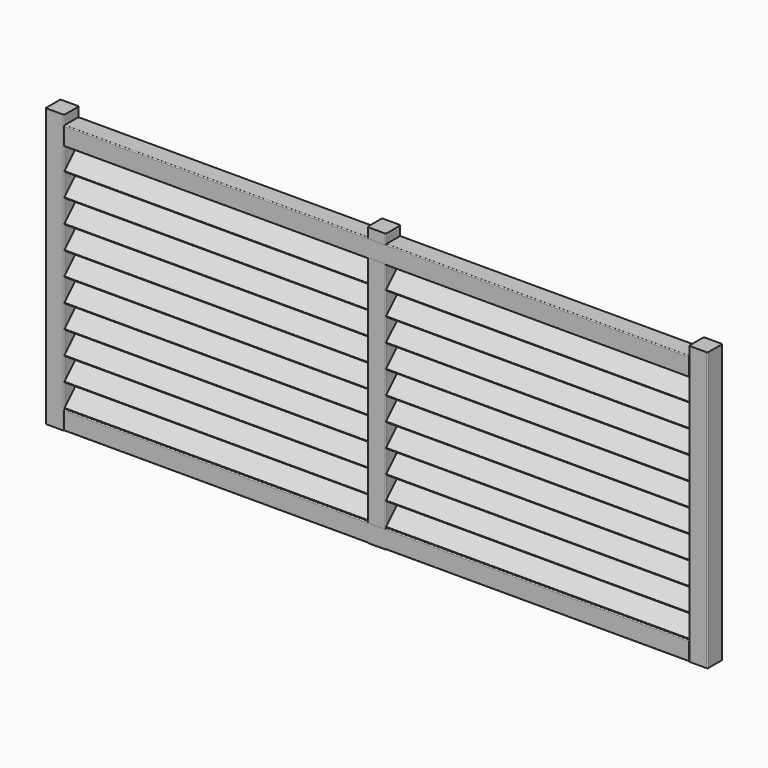
from build123d import *

# Parameters (mm, degrees)
F1_DEPTH      = 3370
F3_DEPTH      = 1400
F3_DEPTH_BACK = 100
F4_W          = 90
F4_H          = 100
F5_DEPTH      = 3370


# Not quite as in the source:
# - a feature names something its author has since deleted; it is built from what else it names


with BuildPart() as f1:
    # F0 (on Right) → F1 (new body)
    with BuildSketch(Plane.YZ):
        with BuildLine():
            ThreePointArc((-1.4142135624, 1.4142135624), (0, 0.8284271247), (1.4142135624, 1.4142135624))
            Line((1.4142135624, 1.4142135624), (89.8025612107, 89.8025612107))
            ThreePointArc((89.8025612107, 89.8025612107), (90.3883476483, 91.2167747731), (89.8025612107, 92.6309883354))
            Line((89.8025612107, 92.6309883354), (85.5599205236, 96.8736290226))
            ThreePointArc((85.5599205236, 96.8736290226), (84.1457069612, 97.4594154602), (82.7314933988, 96.8736290226))
            Line((82.7314933988, 96.8736290226), (-5.6568542495, 8.4852813742))
            ThreePointArc((-5.6568542495, 8.4852813742), (-6.2426406871, 7.0710678119), (-5.6568542495, 5.6568542495))
            Line((-5.6568542495, 5.6568542495), (-1.4142135624, 1.4142135624))
        make_face()
    extrude(amount=F1_DEPTH)


with BuildPart() as f1b:
    # F0 (on Right) → F1, piece 2 (new body)
    with BuildSketch(Plane.YZ):
        with BuildLine():
            ThreePointArc((-1.4142135624, 126.4142135624), (0, 125.8284271247), (1.4142135624, 126.4142135624))
            Line((1.4142135624, 126.4142135624), (89.8025612107, 214.8025612107))
            ThreePointArc((89.8025612107, 214.8025612107), (90.3883476483, 216.2167747731), (89.8025612107, 217.6309883354))
            Line((89.8025612107, 217.6309883354), (85.5599205236, 221.8736290226))
            ThreePointArc((85.5599205236, 221.8736290226), (84.1457069612, 222.4594154602), (82.7314933988, 221.8736290226))
            Line((82.7314933988, 221.8736290226), (-5.6568542495, 133.4852813742))
            ThreePointArc((-5.6568542495, 133.4852813742), (-6.2426406871, 132.0710678119), (-5.6568542495, 130.6568542495))
            Line((-5.6568542495, 130.6568542495), (-1.4142135624, 126.4142135624))
        make_face()
    extrude(amount=F1_DEPTH)


with BuildPart() as f1c:
    # F0 (on Right) → F1, piece 3 (new body)
    with BuildSketch(Plane.YZ):
        with BuildLine():
            ThreePointArc((-1.4142135624, 251.4142135624), (0, 250.8284271247), (1.4142135624, 251.4142135624))
            Line((1.4142135624, 251.4142135624), (89.8025612107, 339.8025612107))
            ThreePointArc((89.8025612107, 339.8025612107), (90.3883476483, 341.2167747731), (89.8025612107, 342.6309883354))
            Line((89.8025612107, 342.6309883354), (85.5599205236, 346.8736290226))
            ThreePointArc((85.5599205236, 346.8736290226), (84.1457069612, 347.4594154602), (82.7314933988, 346.8736290226))
            Line((82.7314933988, 346.8736290226), (-5.6568542495, 258.4852813742))
            ThreePointArc((-5.6568542495, 258.4852813742), (-6.2426406871, 257.0710678119), (-5.6568542495, 255.6568542495))
            Line((-5.6568542495, 255.6568542495), (-1.4142135624, 251.4142135624))
        make_face()
    extrude(amount=F1_DEPTH)


with BuildPart() as f1d:
    # F0 (on Right) → F1, piece 4 (new body)
    with BuildSketch(Plane.YZ):
        with BuildLine():
            ThreePointArc((-1.4142135624, 376.4142135624), (0, 375.8284271247), (1.4142135624, 376.4142135624))
            Line((1.4142135624, 376.4142135624), (89.8025612107, 464.8025612107))
            ThreePointArc((89.8025612107, 464.8025612107), (90.3883476483, 466.2167747731), (89.8025612107, 467.6309883354))
            Line((89.8025612107, 467.6309883354), (85.5599205236, 471.8736290226))
            ThreePointArc((85.5599205236, 471.8736290226), (84.1457069612, 472.4594154602), (82.7314933988, 471.8736290226))
            Line((82.7314933988, 471.8736290226), (-5.6568542495, 383.4852813742))
            ThreePointArc((-5.6568542495, 383.4852813742), (-6.2426406871, 382.0710678119), (-5.6568542495, 380.6568542495))
            Line((-5.6568542495, 380.6568542495), (-1.4142135624, 376.4142135624))
        make_face()
    extrude(amount=F1_DEPTH)


with BuildPart() as f1e:
    # F0 (on Right) → F1, piece 5 (new body)
    with BuildSketch(Plane.YZ):
        with BuildLine():
            ThreePointArc((-1.4142135624, 501.4142135624), (0, 500.8284271247), (1.4142135624, 501.4142135624))
            Line((1.4142135624, 501.4142135624), (89.8025612107, 589.8025612107))
            ThreePointArc((89.8025612107, 589.8025612107), (90.3883476483, 591.2167747731), (89.8025612107, 592.6309883354))
            Line((89.8025612107, 592.6309883354), (85.5599205236, 596.8736290226))
            ThreePointArc((85.5599205236, 596.8736290226), (84.1457069612, 597.4594154602), (82.7314933988, 596.8736290226))
            Line((82.7314933988, 596.8736290226), (-5.6568542495, 508.4852813742))
            ThreePointArc((-5.6568542495, 508.4852813742), (-6.2426406871, 507.0710678119), (-5.6568542495, 505.6568542495))
            Line((-5.6568542495, 505.6568542495), (-1.4142135624, 501.4142135624))
        make_face()
    extrude(amount=F1_DEPTH)


with BuildPart() as f1f:
    # F0 (on Right) → F1, piece 6 (new body)
    with BuildSketch(Plane.YZ):
        with BuildLine():
            ThreePointArc((-1.4142135624, 626.4142135624), (0, 625.8284271247), (1.4142135624, 626.4142135624))
            Line((1.4142135624, 626.4142135624), (89.8025612107, 714.8025612107))
            ThreePointArc((89.8025612107, 714.8025612107), (90.3883476483, 716.2167747731), (89.8025612107, 717.6309883354))
            Line((89.8025612107, 717.6309883354), (85.5599205236, 721.8736290226))
            ThreePointArc((85.5599205236, 721.8736290226), (84.1457069612, 722.4594154602), (82.7314933988, 721.8736290226))
            Line((82.7314933988, 721.8736290226), (-5.6568542495, 633.4852813742))
            ThreePointArc((-5.6568542495, 633.4852813742), (-6.2426406871, 632.0710678119), (-5.6568542495, 630.6568542495))
            Line((-5.6568542495, 630.6568542495), (-1.4142135624, 626.4142135624))
        make_face()
    extrude(amount=F1_DEPTH)


with BuildPart() as f1g:
    # F0 (on Right) → F1, piece 7 (new body)
    with BuildSketch(Plane.YZ):
        with BuildLine():
            ThreePointArc((-1.4142135624, 751.4142135624), (0, 750.8284271247), (1.4142135624, 751.4142135624))
            Line((1.4142135624, 751.4142135624), (89.8025612107, 839.8025612107))
            ThreePointArc((89.8025612107, 839.8025612107), (90.3883476483, 841.2167747731), (89.8025612107, 842.6309883354))
            Line((89.8025612107, 842.6309883354), (85.5599205236, 846.8736290226))
            ThreePointArc((85.5599205236, 846.8736290226), (84.1457069612, 847.4594154602), (82.7314933988, 846.8736290226))
            Line((82.7314933988, 846.8736290226), (-5.6568542495, 758.4852813742))
            ThreePointArc((-5.6568542495, 758.4852813742), (-6.2426406871, 757.0710678119), (-5.6568542495, 755.6568542495))
            Line((-5.6568542495, 755.6568542495), (-1.4142135624, 751.4142135624))
        make_face()
    extrude(amount=F1_DEPTH)


with BuildPart() as f1h:
    # F0 (on Right) → F1, piece 8 (new body)
    with BuildSketch(Plane.YZ):
        with BuildLine():
            ThreePointArc((-1.4142135624, 876.4142135624), (0, 875.8284271247), (1.4142135624, 876.4142135624))
            Line((1.4142135624, 876.4142135624), (89.8025612107, 964.8025612107))
            ThreePointArc((89.8025612107, 964.8025612107), (90.3883476483, 966.2167747731), (89.8025612107, 967.6309883354))
            Line((89.8025612107, 967.6309883354), (85.5599205236, 971.8736290226))
            ThreePointArc((85.5599205236, 971.8736290226), (84.1457069612, 972.4594154602), (82.7314933988, 971.8736290226))
            Line((82.7314933988, 971.8736290226), (-5.6568542495, 883.4852813742))
            ThreePointArc((-5.6568542495, 883.4852813742), (-6.2426406871, 882.0710678119), (-5.6568542495, 880.6568542495))
            Line((-5.6568542495, 880.6568542495), (-1.4142135624, 876.4142135624))
        make_face()
    extrude(amount=F1_DEPTH)


with BuildPart() as f1i:
    # F0 (on Right) → F1, piece 9 (new body)
    with BuildSketch(Plane.YZ):
        with BuildLine():
            ThreePointArc((-1.4142135624, 1001.4142135624), (0, 1000.8284271247), (1.4142135624, 1001.4142135624))
            Line((1.4142135624, 1001.4142135624), (89.8025612107, 1089.8025612107))
            ThreePointArc((89.8025612107, 1089.8025612107), (90.3883476483, 1091.2167747731), (89.8025612107, 1092.6309883354))
            Line((89.8025612107, 1092.6309883354), (85.5599205236, 1096.8736290226))
            ThreePointArc((85.5599205236, 1096.8736290226), (84.1457069612, 1097.4594154602), (82.7314933988, 1096.8736290226))
            Line((82.7314933988, 1096.8736290226), (-5.6568542495, 1008.4852813742))
            ThreePointArc((-5.6568542495, 1008.4852813742), (-6.2426406871, 1007.0710678119), (-5.6568542495, 1005.6568542495))
            Line((-5.6568542495, 1005.6568542495), (-1.4142135624, 1001.4142135624))
        make_face()
    extrude(amount=F1_DEPTH)


with BuildPart() as f1j:
    # F0 (on Right) → F1, piece 10 (new body)
    with BuildSketch(Plane.YZ):
        with BuildLine():
            ThreePointArc((-1.4142135624, 1126.4142135624), (0, 1125.8284271247), (1.4142135624, 1126.4142135624))
            Line((1.4142135624, 1126.4142135624), (89.8025612107, 1214.8025612107))
            ThreePointArc((89.8025612107, 1214.8025612107), (90.3883476483, 1216.2167747731), (89.8025612107, 1217.6309883354))
            Line((89.8025612107, 1217.6309883354), (85.5599205236, 1221.8736290226))
            ThreePointArc((85.5599205236, 1221.8736290226), (84.1457069612, 1222.4594154602), (82.7314933988, 1221.8736290226))
            Line((82.7314933988, 1221.8736290226), (-5.6568542495, 1133.4852813742))
            ThreePointArc((-5.6568542495, 1133.4852813742), (-6.2426406871, 1132.0710678119), (-5.6568542495, 1130.6568542495))
            Line((-5.6568542495, 1130.6568542495), (-1.4142135624, 1126.4142135624))
        make_face()
    extrude(amount=F1_DEPTH)


with BuildPart() as f3:
    # F2 (on Top) → F3 (new body, two sides)
    with BuildSketch(Plane.XY) as f3_sk:
        with BuildLine():
            Line((-95, -8), (-5, -8))
            ThreePointArc((-5, -8), (-1.4644660941, -6.5355339059), (0, -3))
            Line((0, -3), (0, 87))
            ThreePointArc((0, 87), (-1.4644660941, 90.5355339059), (-5, 92))
            Line((-5, 92), (-95, 92))
            ThreePointArc((-95, 92), (-98.5355339059, 90.5355339059), (-100, 87))
            Line((-100, 87), (-100, -3))
            ThreePointArc((-100, -3), (-98.5355339059, -6.5355339059), (-95, -8))
        make_face()
    extrude(amount=F3_DEPTH)
    extrude(f3_sk.sketch, amount=-F3_DEPTH_BACK)


with BuildPart() as f3b:
    # F2 (on Top) → F3, piece 2 (new body, two sides)
    with BuildSketch(Plane.XY) as f3_2_sk:
        with BuildLine():
            Line((1635, 87), (1635, -3))
            ThreePointArc((1635, -3), (1636.4644660941, -6.5355339059), (1640, -8))
            Line((1640, -8), (1730, -8))
            ThreePointArc((1730, -8), (1733.5355339059, -6.5355339059), (1735, -3))
            Line((1735, -3), (1735, 87))
            ThreePointArc((1735, 87), (1733.5355339059, 90.5355339059), (1730, 92))
            Line((1730, 92), (1640, 92))
            ThreePointArc((1640, 92), (1636.4644660941, 90.5355339059), (1635, 87))
        make_face()
    extrude(amount=F3_DEPTH)
    extrude(f3_2_sk.sketch, amount=-F3_DEPTH_BACK)


with BuildPart() as f3c:
    # F2 (on Top) → F3, piece 3 (new body, two sides)
    with BuildSketch(Plane.XY) as f3_3_sk:
        with BuildLine():
            Line((3370, 87), (3370, -3))
            ThreePointArc((3370, -3), (3371.4644660941, -6.5355339059), (3375, -8))
            Line((3375, -8), (3465, -8))
            ThreePointArc((3465, -8), (3468.5355339059, -6.5355339059), (3470, -3))
            Line((3470, -3), (3470, 87))
            ThreePointArc((3470, 87), (3468.5355339059, 90.5355339059), (3465, 92))
            Line((3465, 92), (3375, 92))
            ThreePointArc((3375, 92), (3371.4644660941, 90.5355339059), (3370, 87))
        make_face()
    extrude(amount=F3_DEPTH)
    extrude(f3_3_sk.sketch, amount=-F3_DEPTH_BACK)


with BuildPart() as f5:
    # F4 (on face) → F5 (new body)
    with BuildSketch(Plane.YZ):
        with Locations((42, 1300)):
            Rectangle(F4_W, F4_H)
        with BuildLine():
            Line((87, 1350), (87, 1250))
            ThreePointArc((87, 1250), (90.5355339059, 1251.4644660941), (92, 1255))
            Line((92, 1255), (92, 1345))
            ThreePointArc((92, 1345), (90.5355339059, 1348.5355339059), (87, 1350))
        make_face()
        with BuildLine():
            ThreePointArc((-8, 1255), (-6.5355339059, 1251.4644660941), (-3, 1250))
            Line((-3, 1250), (-3, 1350))
            ThreePointArc((-3, 1350), (-6.5355339059, 1348.5355339059), (-8, 1345))
            Line((-8, 1345), (-8, 1255))
        make_face()
    extrude(amount=F5_DEPTH)


with BuildPart() as f5b:
    # F4 (on face) → F5, piece 2 (new body)
    with BuildSketch(Plane.YZ):
        with Locations((42, -50)):
            Rectangle(F4_W, F4_H)
        with BuildLine():
            Line((87, 0), (87, -100))
            ThreePointArc((87, -100), (90.5355339059, -98.5355339059), (92, -95))
            Line((92, -95), (92, -5))
            ThreePointArc((92, -5), (90.5355339059, -1.4644660941), (87, 0))
        make_face()
        with BuildLine():
            ThreePointArc((-8, -95), (-6.5355339059, -98.5355339059), (-3, -100))
            Line((-3, -100), (-3, 0))
            ThreePointArc((-3, 0), (-6.5355339059, -1.4644660941), (-8, -5))
            Line((-8, -5), (-8, -95))
        make_face()
    extrude(amount=F5_DEPTH)


solid = Compound([f1.part, f1b.part, f1c.part, f1d.part, f1e.part, f1f.part, f1g.part, f1h.part, f1i.part, f1j.part, f3.part, f3b.part, f3c.part, f5.part, f5b.part])
